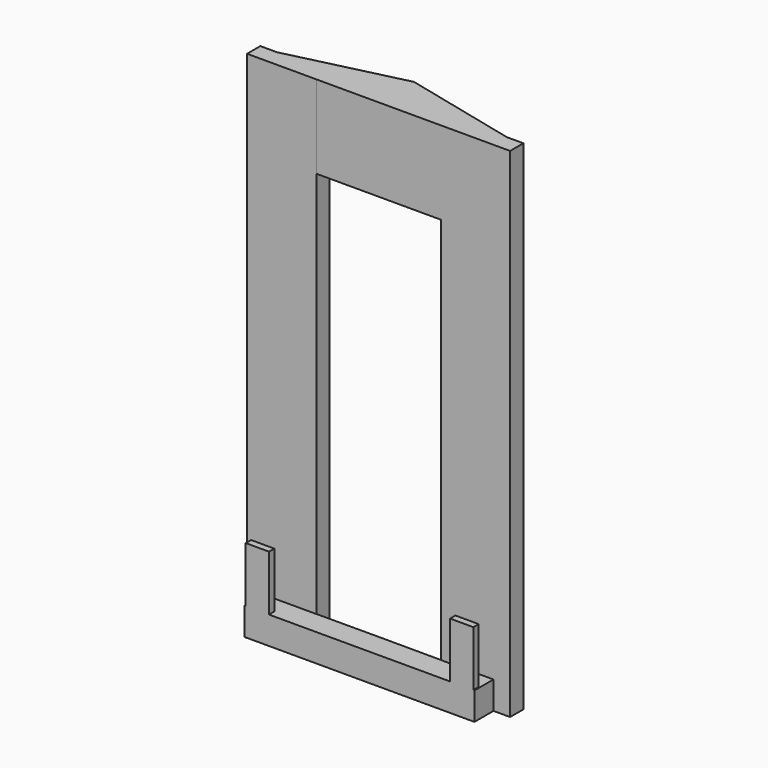
from build123d import *

# Parameters (mm, degrees)
F0_W      = 4.2
F0_H      = 1.2
F1_DEPTH  = 15
F0_W_2    = 32.7
F2_DEPTH  = 5
F4_DEPTH  = 5
F6_DEPTH  = 5
F7_W      = 9.5
F7_H      = 3
F8_DEPTH  = 90
F9_W      = 9.5
F9_H      = 3
F10_DEPTH = 15
F11_DEPTH = 10.1
F12_DEPTH = 5
F13_W     = 5
F13_H     = 5.1
F14_DEPTH = 4.5
F15_W     = 3
F15_H     = 3
F16_DEPTH = 90


with BuildPart() as f1:
    # F0 (on Top) → F1 (new body)
    with BuildSketch(Plane.XY):
        with Locations((-86.9470929563, 1.1125010281)):
            Rectangle(F0_W, F0_H)
    extrude(amount=F1_DEPTH)



with BuildPart() as f1b:
    # F0 (on Top) → F1, piece 2 (new body)
    with BuildSketch(Plane.XY):
        with Locations((-50.0470929563, 1.1125010281)):
            Rectangle(F0_W, F0_H)
    extrude(amount=F1_DEPTH)


with BuildPart() as f1_1:
    add(f1.part)

    add(f1b.part)  # F2 merges F1b
    # F0 (on Top) → F2 (join)
    with BuildSketch(Plane.XY):
        with Locations((-68.4970929563, 1.1125010281)):
            Rectangle(F0_W_2, F0_H)
    extrude(amount=F2_DEPTH)

    # F3 (on face) → F4 (join)
    with BuildSketch(Plane(origin=(0, 0, 0), x_dir=(1, 0, 0), z_dir=(0, 0, -1))):
        Polygon((-52.1470929563, -0.5125010281), (-84.8470929563, -0.5125010281), (-89.2470929563, -0.5125010281), (-89.2470929563, -4.8120530977), (-68.4970929563, -4.8593617954), (-47.7470929563, -4.8125010281), (-47.7470929563, -0.5125010281), align=None)
    extrude(amount=-F4_DEPTH)

    # F5: union 

    # F3 (on face) → F6 (join)
    with BuildSketch(Plane(origin=(0, 0, 0), x_dir=(1, 0, 0), z_dir=(0, 0, -1))):
        Polygon((-52.1470929563, -0.5125010281), (-84.8470929563, -0.5125010281), (-89.2470929563, -0.5125010281), (-89.2470929563, -4.8120530977), (-68.4970929563, -4.8593617954), (-47.7470929563, -4.8125010281), (-47.7470929563, -0.5125010281), align=None)
    extrude(amount=-F6_DEPTH)

    # F7 (on face) → F8 (join)
    with BuildSketch(Plane(origin=(0, 0, 0), x_dir=(1, 0, 0), z_dir=(0, 0, -1))):
        with Locations((-84.4970929563, -6.3120530977)):
            Rectangle(F7_W, F7_H)
        with Locations((-52.4970929563, -6.3125010281)):
            Rectangle(F7_W, F7_H)
    extrude(amount=-F8_DEPTH)

    # F9 (on face) → F10 (join)
    with BuildSketch(Plane.XY.offset(90)):
        Polygon((-89.2470929563, 4.8125010281), (-57.2470929563, 4.8125010281), (-57.2470929563, 7.8125010281), (-68.4970929563, 7.8125010281), (-89.2470929563, 7.8125010281), align=None)
        with Locations((-52.4970929563, 6.3125010281)):
            Rectangle(F9_W, F9_H)
        Polygon((-57.2470929563, 7.8125010281), (-47.7470929563, 7.8125010281), (-65.9970929563, 12.2100913895), (-65.9970929563, 10.3125010281), (-68.4970929563, 10.3125010281), (-68.4970929563, 7.8125010281), align=None)
        Polygon((-70.9970929563, 12.2100913895), (-89.2470929563, 7.8125010281), (-68.4970929563, 7.8125010281), (-68.4970929563, 10.3125010281), (-70.9970929563, 10.3125010281), align=None)
        Polygon((-68.4970929563, 10.3125010281), (-68.4970929563, 12.8125010281), (-70.9970929563, 12.2100913895), (-70.9970929563, 10.3125010281), align=None)
        Polygon((-65.9970929563, 10.3125010281), (-65.9970929563, 12.2100913895), (-68.4970929563, 12.8125010281), (-68.4970929563, 10.3125010281), align=None)
    extrude(amount=-F10_DEPTH)

    # F9 (on face) → F11 (cut)
    with BuildSketch(Plane.XY.offset(90)):
        Polygon((-68.4970929563, 10.3125010281), (-68.4970929563, 12.8125010281), (-70.9970929563, 12.2100913895), (-70.9970929563, 10.3125010281), align=None)
        Polygon((-65.9970929563, 10.3125010281), (-65.9970929563, 12.2100913895), (-68.4970929563, 12.8125010281), (-68.4970929563, 10.3125010281), align=None)
    extrude(amount=-F11_DEPTH, mode=Mode.SUBTRACT)

    # F9 (on face) → F12 (join)
    with BuildSketch(Plane.XY.offset(90)):
        Polygon((-65.9970929563, 10.3125010281), (-65.9970929563, 12.2100913895), (-68.4970929563, 12.8125010281), (-68.4970929563, 10.3125010281), align=None)
        Polygon((-68.4970929563, 10.3125010281), (-68.4970929563, 12.8125010281), (-70.9970929563, 12.2100913895), (-70.9970929563, 10.3125010281), align=None)
    extrude(amount=-F12_DEPTH)

    # F13 (on face) → F14 (cut)
    with BuildSketch(Plane(origin=(0, 10.3125010281, 0), x_dir=(-1, 0, 0), z_dir=(0, 1, 0))):
        with Locations((68.4970929563, 82.45)):
            Rectangle(F13_W, F13_H)
    extrude(amount=-F14_DEPTH, mode=Mode.SUBTRACT)

    # F15 (on face) → F16 (join)
    with BuildSketch(Plane(origin=(0, 0, 0), x_dir=(1, 0, 0), z_dir=(0, 0, -1))):
        with Locations((-46.2470929563, -6.3125010281)):
            Rectangle(F15_W, F15_H)
        with Locations((-90.7470929563, -6.3120530977)):
            Rectangle(F15_W, F15_H)
    extrude(amount=-F16_DEPTH)


solid = f1_1.part
